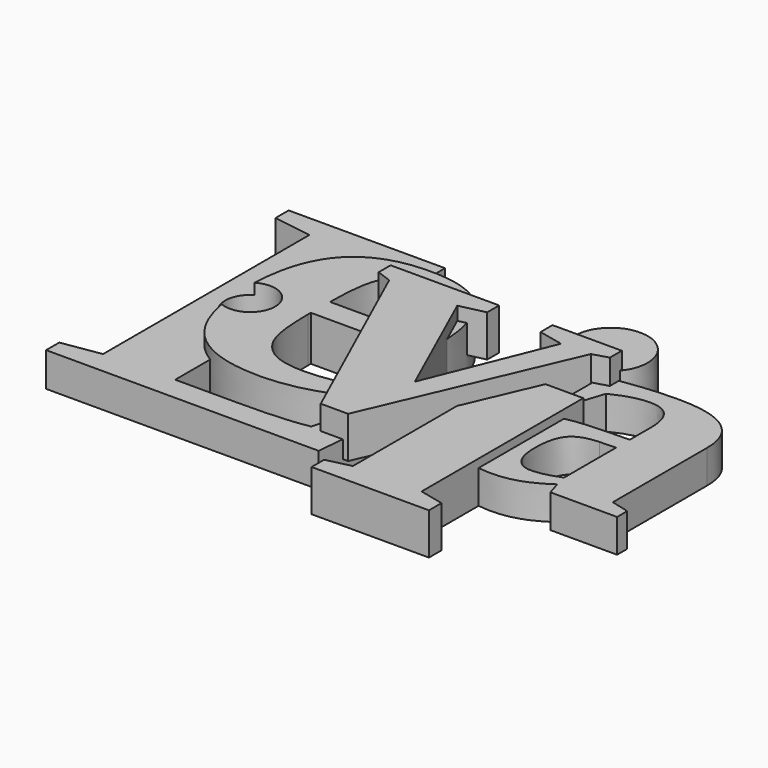
from build123d import *

# Parameters (mm, degrees)
F0_TEXT_SIZE = 27.7777777778
F1_DEPTH     = 2.05
F2_TEXT_SIZE = 27.7777777778
F3_DEPTH     = 2.7
F5_START     = 1
F4_TEXT_SIZE = 27.7777777778
F5_DEPTH     = 2.5
F6_TEXT_SIZE = 29.2393301303
F7_DEPTH     = 2.5
F8_TEXT_SIZE = 23.7164501515
F9_DEPTH     = 2
F10_R        = 1.5
F11_DEPTH    = 2.7010001


# Not quite as in the source:
# - Text() gives the source's letters only with a copy of the font that has no kerning and outlines rounded to 1/6400 em; it was checked with that copy


with BuildPart() as f1:
    # F0 (on Top) → F1 (new body)
    with BuildSketch(Plane.XY):
        with Locations((-20.4139200507, -1.7214124091)):
            Text('L', F0_TEXT_SIZE, font='Tinos', font_style=FontStyle.BOLD, text_align=(TextAlign.LEFT, TextAlign.BOTTOM))
    extrude(amount=F1_DEPTH)

    # F2 (on Top) → F3 (join)
    with BuildSketch(Plane.XY):
        with Locations((-16.7590333404, 1.7585136193)):
            Text('e', F2_TEXT_SIZE, font='Tinos', font_style=FontStyle.BOLD, text_align=(TextAlign.LEFT, TextAlign.BOTTOM))
    extrude(amount=F3_DEPTH)

    # F4 (on Top) → F5 (join)
    with BuildSketch(Plane.XY.offset(F5_START)):
        with Locations((-10.9649912924, 0.1747674377)):
            Text('v', F4_TEXT_SIZE, font='Tinos', font_style=FontStyle.BOLD, text_align=(TextAlign.LEFT, TextAlign.BOTTOM))
    extrude(amount=F5_DEPTH)

    # F6 (on Top) → F7 (join)
    with BuildSketch(Plane.XY):
        with Locations((-2.9061324894, -3.8852933794)):
            Text('i', F6_TEXT_SIZE, font='Tinos', font_style=FontStyle.BOLD, text_align=(TextAlign.LEFT, TextAlign.BOTTOM))
    extrude(amount=F7_DEPTH)

    # F8 (on Top) → F9 (join)
    with BuildSketch(Plane.XY):
        with Locations((0, 1.8523000181)):
            Text('a', F8_TEXT_SIZE, font='Tinos', font_style=FontStyle.BOLD, text_align=(TextAlign.LEFT, TextAlign.BOTTOM))
    extrude(amount=F9_DEPTH)

    # F10 (on face) → F11 (cut, through all)
    with BuildSketch(Plane.XY.offset(2.7)):
        with Locations((-15.0321479887, 7.4697330128)):
            Circle(F10_R)
    extrude(amount=-F11_DEPTH, mode=Mode.SUBTRACT)


solid = f1.part
